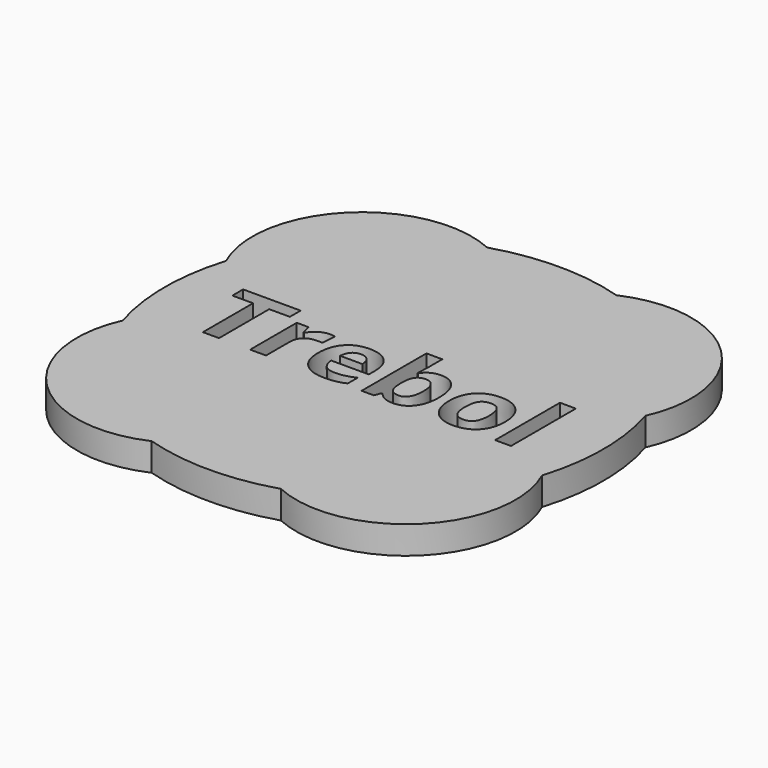
from build123d import *

# Parameters (mm, degrees)
F1_DEPTH     = 25.4
F2_TEXT_SIZE = 97.2222222222
F3_DEPTH     = 25.4


# Not quite as in the source:
# - Text() gives the source's letters only with a copy of the font that has no kerning and outlines rounded to 1/6400 em; it was checked with that copy


with BuildPart() as f1:
    # F0 (on Top) → F1 (new body)
    with BuildSketch(Plane.XY):
        with BuildLine():
            ThreePointArc((-58.8562172234, 191.1437827766), (-170.7106781187, 170.7106781187), (-191.1437827766, 58.8562172234))
            ThreePointArc((-191.1437827766, 58.8562172234), (-200, 0), (-191.1437827766, -58.8562172234))
            ThreePointArc((-191.1437827766, -58.8562172234), (-170.7106781187, -170.7106781187), (-58.8562172234, -191.1437827766))
            ThreePointArc((-58.8562172234, -191.1437827766), (0, -200), (58.8562172234, -191.1437827766))
            ThreePointArc((58.8562172234, -191.1437827766), (170.7106781187, -170.7106781187), (191.1437827766, -58.8562172234))
            ThreePointArc((191.1437827766, -58.8562172234), (200, 0), (191.1437827766, 58.8562172234))
            ThreePointArc((191.1437827766, 58.8562172234), (170.7106781187, 170.7106781187), (58.8562172234, 191.1437827766))
            ThreePointArc((58.8562172234, 191.1437827766), (0, 200), (-58.8562172234, 191.1437827766))
        make_face()
    extrude(amount=F1_DEPTH)

    # F2 (on face) → F3 (cut)
    with BuildSketch(Plane.XY.offset(25.4)):
        with Locations((-156.1538547541, -37.2028046097)):
            Text('Trebol', F2_TEXT_SIZE, font='Open Sans', font_style=FontStyle.BOLD, text_align=(TextAlign.LEFT, TextAlign.BOTTOM))
    extrude(amount=-F3_DEPTH, mode=Mode.SUBTRACT)


solid = f1.part
